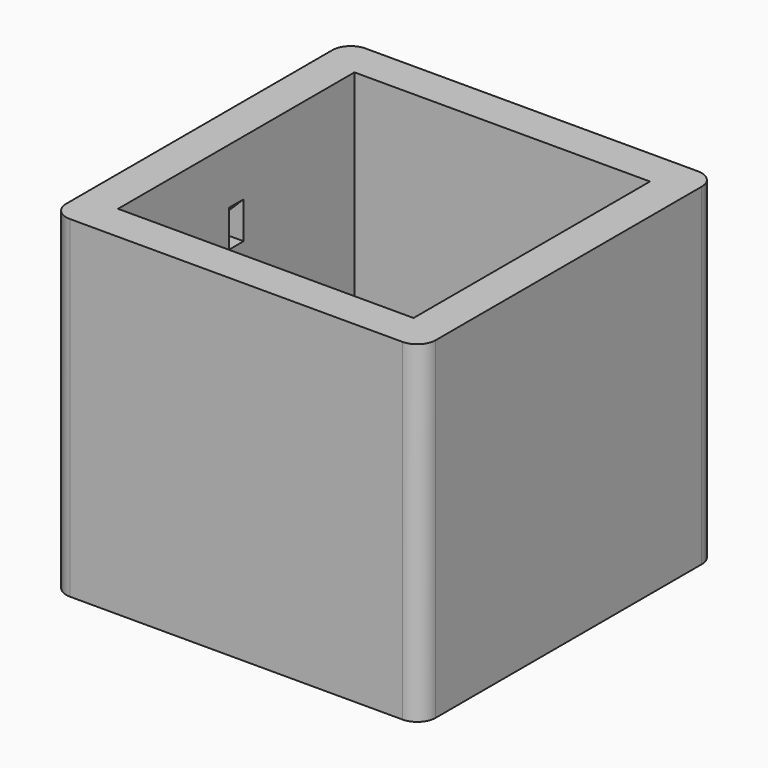
from build123d import *

# Parameters (mm, degrees)
F0_W     = 20.32
F0_H     = 20.32
F1_DEPTH = 2.54
F0_W_2   = 25.4
F0_H_2   = 25.4
F2_DEPTH = 22.86
F3_W     = 1.27
F3_H     = 2.54
F3_W_2   = 0.635
F3_H_2   = 1.27
F4_DEPTH = 1.27
F5_SIZE  = 1.26999
F6_W     = 1.27
F6_H     = 2.54
F7_DEPTH = 1.27
F8_SIZE  = 1.26999
F9_R     = 1.27


# Not quite as in the source:
# - a fillet or chamfer is up to 0.001 mm smaller than in the source, because OpenCascade refuses the exact size


with BuildPart() as f1:
    # F0 (on Top) → F1 (new body)
    with BuildSketch(Plane.XY):
        Rectangle(F0_W, F0_H)
    extrude(amount=F1_DEPTH)

    # F0 (on Top) → F2 (join)
    with BuildSketch(Plane.XY):
        Rectangle(F0_W_2, F0_H_2)
        Rectangle(F0_W, F0_H, mode=Mode.SUBTRACT)
    extrude(amount=F2_DEPTH)

    # F3 (on face) → F4 (cut)
    with BuildSketch(Plane.YZ.offset(-10.16)):
        with Locations((0, 17.78)):
            Rectangle(F3_W, F3_H)
        with Locations((0, 17.78)):
            Rectangle(F3_W_2, F3_H_2, mode=Mode.SUBTRACT)
        with Locations((0, 17.78)):
            Rectangle(F3_W_2, F3_H_2)
    extrude(amount=-F4_DEPTH, mode=Mode.SUBTRACT)

    # F5 (size 1.27 in the source; OpenCascade refuses exactly that, so slightly less here)
    f5_edges = [f1.edges().sort_by_distance(p)[0] for p in [
        (-11.43, 0, 19.05),
    ]]
    chamfer(f5_edges, length=F5_SIZE)

    # F6 (on face) → F7 (cut)
    with BuildSketch(Plane(origin=(10.16, 0, 0), x_dir=(0, -1, 0), z_dir=(-1, 0, 0))):
        with Locations((0, 17.78)):
            Rectangle(F6_W, F6_H)
    extrude(amount=-F7_DEPTH, mode=Mode.SUBTRACT)

    # F8 (size 1.27 in the source; OpenCascade refuses exactly that, so slightly less here)
    f8_edges = [f1.edges().sort_by_distance(p)[0] for p in [
        (11.43, 0, 19.05),
    ]]
    chamfer(f8_edges, length=F8_SIZE)

    # F9
    f9_edges = [f1.edges().sort_by_distance(p)[0] for p in [
        (-12.7, -12.7, 11.43),
        (12.7, -12.7, 11.43),
        (12.7, 12.7, 11.43),
        (-12.7, 12.7, 11.43),
    ]]
    fillet(f9_edges, radius=F9_R)


solid = f1.part
